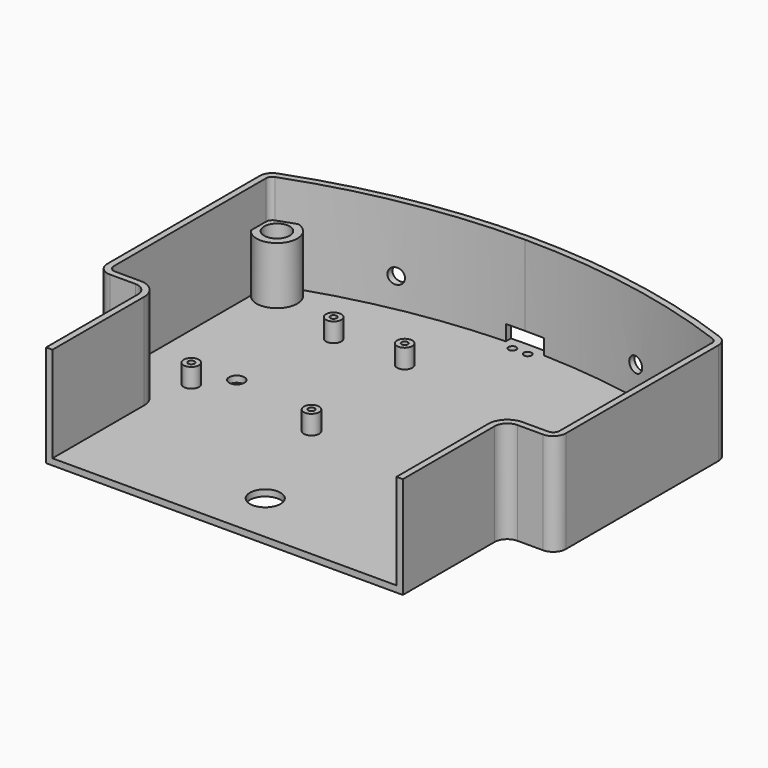
from build123d import *

# Parameters (mm, degrees)
F1_DEPTH  = 40
F2_W      = 100
F2_H      = 200
F3_DEPTH  = 100
F4_R      = 5
F5_T      = -2.5
F6_R      = 6
F7_DEPTH  = 25
F8_R      = 3
F9_DEPTH  = 25
F10_R     = 8
F11_DEPTH = 25
F12_R     = 5
F13_DEPTH = 25
F14_R     = 3
F14_R_2   = 1.25
F15_DEPTH = 10
F16_R     = 3
F17_DEPTH = 150
F18_W     = 15
F18_H     = 6
F19_DEPTH = 250
F20_R     = 1.5
F21_DEPTH = 12.5


with BuildPart() as f1:
    # F0 (on Top) → F1 (new body)
    with BuildSketch(Plane.XY):
        with BuildLine():
            Line((-90, 83.2380757938), (-90, -50))
            Line((-90, -50), (90, -50))
            Line((90, -50), (90, 83.2380757938))
            ThreePointArc((90, 83.2380757938), (45.7737973711, 95.7737973711), (0, 100))
            ThreePointArc((0, 100), (-45.7737973711, 95.7737973711), (-90, 83.2380757938))
        make_face()
    extrude(amount=F1_DEPTH)

    # F2 (on Top) → F3 (cut)
    with BuildSketch(Plane.XY):
        with Locations((-120, -100)):
            Rectangle(F2_W, F2_H)
        with Locations((120, -100)):
            Rectangle(F2_W, F2_H)
    extrude(amount=F3_DEPTH, mode=Mode.SUBTRACT)

    # F4
    f4_edges = [f1.edges().sort_by_distance(p)[0] for p in [
        (-90, 83.238076, 20),
        (90, 83.238076, 20),
        (90, 0, 20),
        (70, 0, 20),
        (-90, 0, 20),
        (-70, 0, 20),
    ]]
    fillet(f4_edges, radius=F4_R)

    # F5
    f5_openings = [f1.faces().sort_by_distance(p)[0] for p in [
        (0, 26.262097, 40),
        (0, -50, 20),
    ]]
    offset(amount=F5_T, openings=f5_openings)

    # F6 (on Top) → F7 (cut)
    with BuildSketch(Plane.XY):
        with Locations((0, -30)):
            Circle(F6_R)
    extrude(amount=F7_DEPTH, mode=Mode.SUBTRACT)

    # F8 (on Top) → F9 (cut)
    with BuildSketch(Plane.XY):
        with Locations((-55.8614357137, 25.8614357137)):
            Circle(F8_R)
        with Locations((55.8614357137, 25.8614357137)):
            Circle(F8_R)
    extrude(amount=F9_DEPTH, mode=Mode.SUBTRACT)

    # F10 (on Top) → F11 (join)
    with BuildSketch(Plane.XY):
        with Locations((-81, 77)):
            Circle(F10_R)
        with Locations((81, 77)):
            Circle(F10_R)
    extrude(amount=F11_DEPTH)

    # F12 (on Top) → F13 (cut)
    with BuildSketch(Plane.XY):
        with Locations((-81, 77)):
            Circle(F12_R)
        with Locations((81, 77)):
            Circle(F12_R)
    extrude(amount=F13_DEPTH, mode=Mode.SUBTRACT)

    # F14 (on Top) → F15 (join)
    with BuildSketch(Plane.XY):
        with Locations((-65, 15)):
            Circle(F14_R)
        with Locations((-65, 15)):
            Circle(F14_R_2, mode=Mode.SUBTRACT)
        with Locations((-49.8, 65.8)):
            Circle(F14_R)
        with Locations((-49.8, 65.8)):
            Circle(F14_R_2, mode=Mode.SUBTRACT)
        with Locations((-21.9, 65.8)):
            Circle(F14_R)
        with Locations((-21.9, 65.8)):
            Circle(F14_R_2, mode=Mode.SUBTRACT)
        with Locations((-16.8, 13.7)):
            Circle(F14_R)
        with Locations((-16.8, 13.7)):
            Circle(F14_R_2, mode=Mode.SUBTRACT)
    extrude(amount=F15_DEPTH)

    # F16 (on Front) → F17 (cut, symmetric)
    with BuildSketch(Plane.XZ):
        with Locations((47, 14)):
            Circle(F16_R)
        with Locations((-47, 14)):
            Circle(F16_R)
    extrude(amount=F17_DEPTH, both=True, mode=Mode.SUBTRACT)

    # F18 (on Front) → F19 (cut)
    with BuildSketch(Plane.XZ):
        with Locations((0, 5.5)):
            Rectangle(F18_W, F18_H)
    extrude(amount=-F19_DEPTH, mode=Mode.SUBTRACT)

    # F20 (on Top) → F21 (cut, symmetric)
    with BuildSketch(Plane.XY):
        with Locations((-3, 95)):
            Circle(F20_R)
        with Locations((3, 95)):
            Circle(F20_R)
    extrude(amount=F21_DEPTH, both=True, mode=Mode.SUBTRACT)


solid = f1.part
